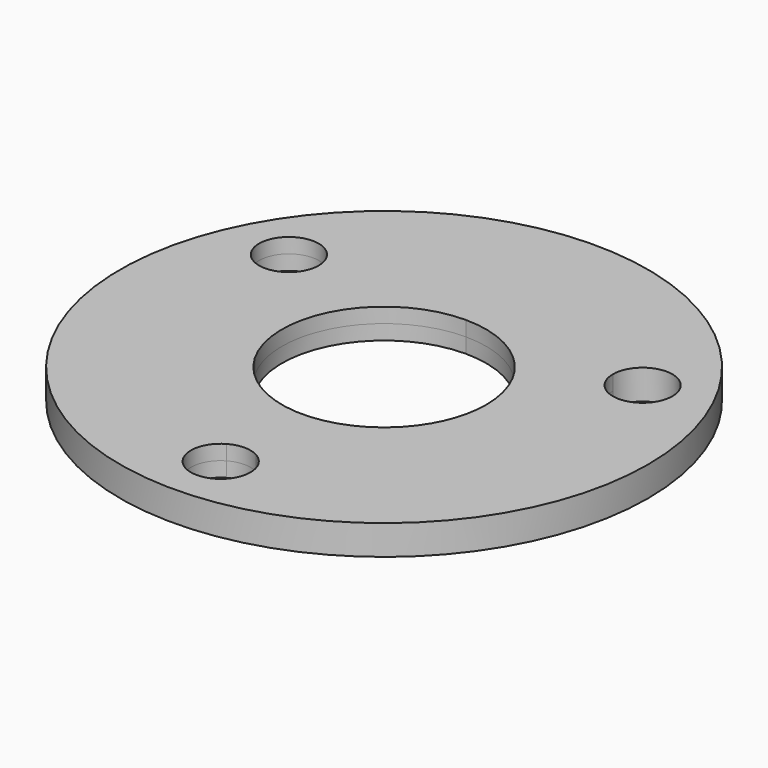
from build123d import *

# Parameters (mm, degrees)
F0_R     = 28.1326878824
F1_DEPTH = 1.5875


with BuildPart() as f1:
    # F0 (on Top) → F1 (new body, symmetric)
    with BuildSketch(Plane.XY):
        Circle(F0_R)
        with BuildLine():
            Line((-15.6764677845, 10.8839), (0, 10.8839))
            Line((0, 10.8839), (15.6764677845, 10.8839))
            ThreePointArc((15.6764677845, 10.8839), (18.8514677845, 14.0589), (22.0264677845, 10.8839))
            ThreePointArc((22.0264677845, 10.8839), (20.4389677845, 8.134269343), (17.2639677845, 8.134269343))
            Line((17.2639677845, 8.134269343), (9.4257339481, -5.4419499033))
            Line((9.4257339481, -5.4419499033), (1.5875, -19.018169343))
            ThreePointArc((1.5875, -19.018169343), (2.749630657, -20.1803), (3.175, -21.7678))
            ThreePointArc((3.175, -21.7678), (-1.5875, -24.517430657), (-1.5875, -19.018169343))
            Line((-1.5875, -19.018169343), (-9.4257338301, -5.4419501077))
            Line((-9.4257338301, -5.4419501077), (-17.2639677845, 8.134269343))
            ThreePointArc((-17.2639677845, 8.134269343), (-21.6010984415, 12.4714), (-15.6764677845, 10.8839))
        make_face(mode=Mode.SUBTRACT)
        with BuildLine():
            ThreePointArc((0, 10.8839), (7.6960794958, 7.6960794958), (10.8839, 0))
            ThreePointArc((10.8839, 0), (10.5130401152, -2.8169605511), (9.4257339481, -5.4419499033))
            Line((9.4257339481, -5.4419499033), (17.2639677845, 8.134269343))
            ThreePointArc((17.2639677845, 8.134269343), (16.1018371275, 9.2964), (15.6764677845, 10.8839))
            Line((15.6764677845, 10.8839), (0, 10.8839))
        make_face()
        with BuildLine():
            ThreePointArc((-9.4257338301, -5.4419501077), (-9.4257339233, 5.4419499462), (0, 10.8839))
            Line((0, 10.8839), (-15.6764677845, 10.8839))
            ThreePointArc((-15.6764677845, 10.8839), (-16.1018371275, 9.2964), (-17.2639677845, 8.134269343))
            Line((-17.2639677845, 8.134269343), (-9.4257338301, -5.4419501077))
        make_face()
        with BuildLine():
            Line((1.5875, -19.018169343), (9.4257339481, -5.4419499033))
            ThreePointArc((9.4257339481, -5.4419499033), (1.18e-07, -10.8839), (-9.4257338301, -5.4419501077))
            Line((-9.4257338301, -5.4419501077), (-1.5875, -19.018169343))
            ThreePointArc((-1.5875, -19.018169343), (0, -18.5928), (1.5875, -19.018169343))
        make_face()
    extrude(amount=F1_DEPTH, both=True)


solid = f1.part
